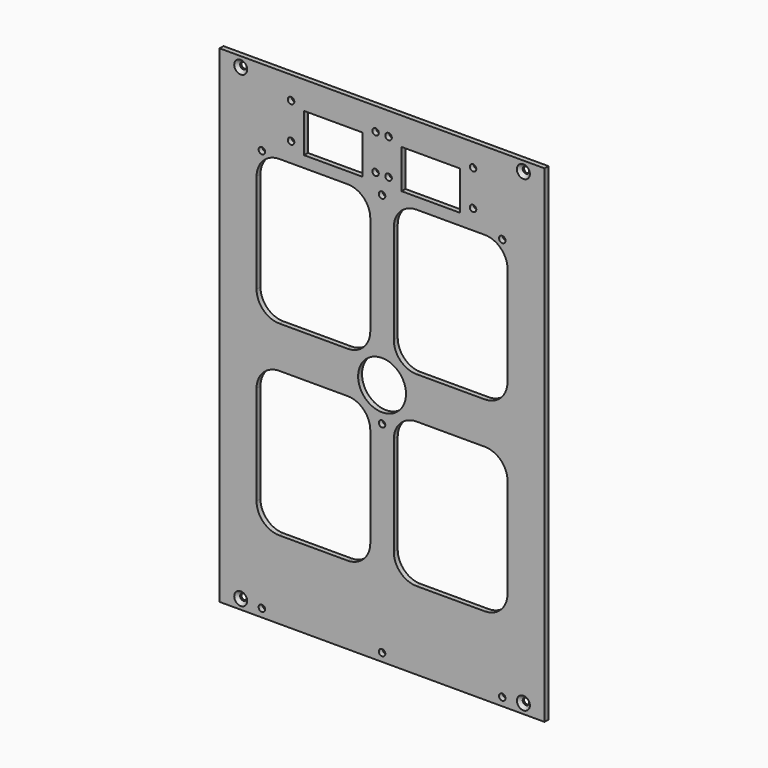
from build123d import *

# Parameters (mm, degrees)
F0_W           = 100
F0_H           = 150
F0_R           = 7.3677826157
F1_DEPTH       = 1.5
F3_D           = 2
F3_CSINK_D     = 4
F3_CSINK_ANGLE = 90
F4_D           = 2
F6_D           = 2


# Not quite as in the source:
# - a feature names something its author has since deleted; it is built from what else it names


with BuildPart() as f1:
    # F0 (on Front) → F1 (new body)
    with BuildSketch(Plane.XZ):
        Rectangle(F0_W, F0_H)
        with BuildLine():
            Line((-31.6183936375, -6.4180564158), (-10.6183936375, -6.4180564158))
            ThreePointArc((-10.6183936375, -6.4180564158), (-5.6686461691, -8.4683089475), (-3.6183936375, -13.4180564158))
            Line((-3.6183936375, -13.4180564158), (-3.6183936375, -44))
            ThreePointArc((-3.6183936375, -44), (-5.6686461691, -48.9497474683), (-10.6183936375, -51))
            Line((-10.6183936375, -51), (-31.6183936375, -51))
            ThreePointArc((-31.6183936375, -51), (-36.5681411058, -48.9497474683), (-38.6183936375, -44))
            Line((-38.6183936375, -44), (-38.6183936375, -13.4180564158))
            ThreePointArc((-38.6183936375, -13.4180564158), (-36.5681411058, -8.4683089475), (-31.6183936375, -6.4180564158))
        make_face(mode=Mode.SUBTRACT)
        with BuildLine():
            ThreePointArc((38.6183936375, -44), (36.5681411058, -48.9497474683), (31.6183936375, -51))
            Line((31.6183936375, -51), (10.6183936375, -51))
            ThreePointArc((10.6183936375, -51), (5.6686461691, -48.9497474683), (3.6183936375, -44))
            Line((3.6183936375, -44), (3.6183936375, -13.4180564158))
            ThreePointArc((3.6183936375, -13.4180564158), (5.6686461691, -8.4683089475), (10.6183936375, -6.4180564158))
            Line((10.6183936375, -6.4180564158), (31.6183936375, -6.4180564158))
            ThreePointArc((31.6183936375, -6.4180564158), (36.5681411058, -8.4683089475), (38.6183936375, -13.4180564158))
            Line((38.6183936375, -13.4180564158), (38.6183936375, -44))
        make_face(mode=Mode.SUBTRACT)
        with BuildLine():
            ThreePointArc((-3.6183936375, 13.4180564158), (-5.6686461691, 8.4683089475), (-10.6183936375, 6.4180564158))
            Line((-10.6183936375, 6.4180564158), (-31.6183936375, 6.4180564158))
            ThreePointArc((-31.6183936375, 6.4180564158), (-36.5681411058, 8.4683089475), (-38.6183936375, 13.4180564158))
            Line((-38.6183936375, 13.4180564158), (-38.6183936375, 44))
            ThreePointArc((-38.6183936375, 44), (-36.5681411058, 48.9497474683), (-31.6183936375, 51))
            Line((-31.6183936375, 51), (-10.6183936375, 51))
            ThreePointArc((-10.6183936375, 51), (-5.6686461691, 48.9497474683), (-3.6183936375, 44))
            Line((-3.6183936375, 44), (-3.6183936375, 13.4180564158))
        make_face(mode=Mode.SUBTRACT)
        Polygon((-24, 54.5), (-24, 66.5), (-15, 66.5), (-6, 66.5), (-6, 54.5), (-15, 54.5), align=None, mode=Mode.SUBTRACT)
        Circle(F0_R, mode=Mode.SUBTRACT)
        with BuildLine():
            ThreePointArc((10.6183936375, 6.4180564158), (5.6686461691, 8.4683089475), (3.6183936375, 13.4180564158))
            Line((3.6183936375, 13.4180564158), (3.6183936375, 44))
            ThreePointArc((3.6183936375, 44), (5.6686461691, 48.9497474683), (10.6183936375, 51))
            Line((10.6183936375, 51), (31.6183936375, 51))
            ThreePointArc((31.6183936375, 51), (36.5681411058, 48.9497474683), (38.6183936375, 44))
            Line((38.6183936375, 44), (38.6183936375, 13.4180564158))
            ThreePointArc((38.6183936375, 13.4180564158), (36.5681411058, 8.4683089475), (31.6183936375, 6.4180564158))
            Line((31.6183936375, 6.4180564158), (10.6183936375, 6.4180564158))
        make_face(mode=Mode.SUBTRACT)
        Polygon((6, 54.5), (6, 66.5), (15, 66.5), (24, 66.5), (24, 54.5), (15, 54.5), align=None, mode=Mode.SUBTRACT)
    extrude(amount=F1_DEPTH)

    # F3 (through all)
    with Locations(Plane.XZ.offset(1.5)):
        with Locations((-43.5, -72), (43.5, -72), (43.5, 72), (-43.5, 72)):
            CounterSinkHole(F3_D / 2, F3_CSINK_D / 2, counter_sink_angle=F3_CSINK_ANGLE)

    # F4 (through all)
    with Locations(Plane(origin=(0, 0, 0), x_dir=(1, 0, 0), z_dir=(0, 1, 0))):
        with Locations((-28, -68), (-28, -57), (-2, -57), (-2, -68), (2, -68), (2, -57), (28, -57), (28, -68)):
            Hole(F4_D / 2)

    # F6 (through all)
    with Locations(Plane(origin=(0, 0, 0), x_dir=(1, 0, 0), z_dir=(0, 1, 0))):
        with Locations((-37, 72.5), (0, 72.5), (37, 72.5), (0, 10.5), (0, -51.5), (37, -51.5), (-37, -51.5)):
            Hole(F6_D / 2)


solid = f1.part
